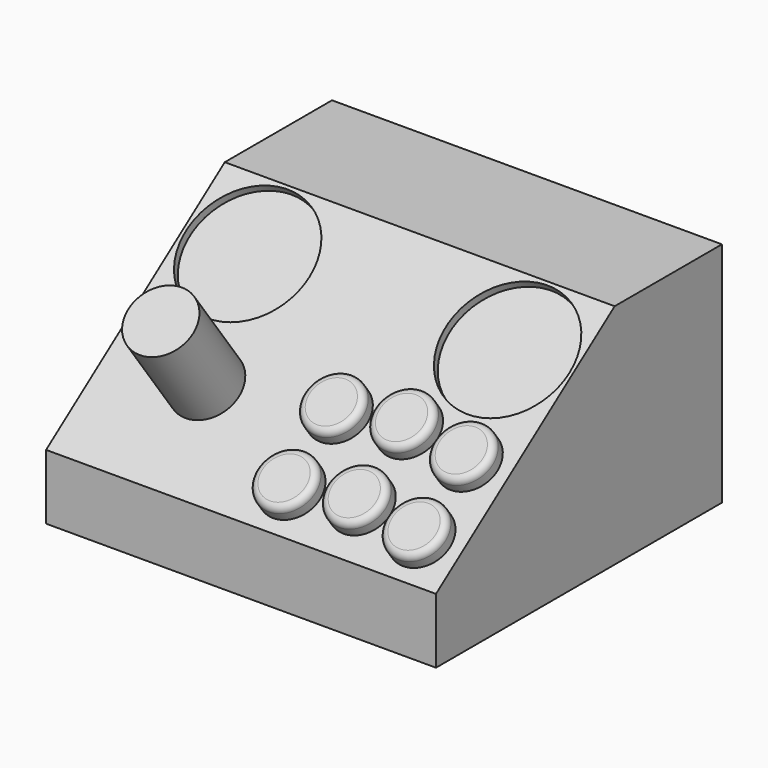
from build123d import *

# Parameters (mm, degrees)
F0_W     = 82.5227291513
F0_H     = 100
F1_DEPTH = 120
F2_R     = 38.1
F3_DEPTH = 5
F4_DEPTH = 5
F2_R_2   = 17.5
F5_DEPTH = 10
F6_DEPTH = 10
F2_R_3   = 20
F7_DEPTH = 60
F8_R     = 4
F9_R     = 4


# Not quite as in the source:
# - the program builds the solid bodies; features that only make, move or delete a surface that nothing else refers to are left out


with BuildPart() as f1:
    # F0 (on Right) → F1 (new body, symmetric)
    with BuildSketch(Plane.YZ):
        Polygon((27.4772708487, -50), (27.4772708487, 50), (-110, -50), align=None)
        with Locations((68.7386354243, 0)):
            Rectangle(F0_W, F0_H)
        Polygon((27.4772708487, -50), (-110, -50), (-110, -90), (110, -90), (110, -50), align=None)
    extrude(amount=F1_DEPTH, both=True)

    # F2 (on face) → F3 (cut)
    with BuildSketch(Plane(origin=(0, -14.2772887805, 19.6280269666), x_dir=(1, 0, 0), z_dir=(0, -0.5882352941, 0.8086898285))):
        with Locations((-80, 11.6323541567)):
            Circle(F2_R)
    extrude(amount=-F3_DEPTH, mode=Mode.SUBTRACT)

    # F2 (on face) → F4 (cut)
    with BuildSketch(Plane(origin=(0, -14.2772887805, 19.6280269666), x_dir=(1, 0, 0), z_dir=(0, -0.5882352941, 0.8086898285))):
        with Locations((80, 11.6323541567)):
            Circle(F2_R)
    extrude(amount=-F4_DEPTH, mode=Mode.SUBTRACT)

    # F2 (on face) → F5 (join)
    with BuildSketch(Plane(origin=(0, -14.2772887805, 19.6280269666), x_dir=(1, 0, 0), z_dir=(0, -0.5882352941, 0.8086898285))):
        with Locations((15, -48.3676458433)):
            Circle(F2_R_2)
    extrude(amount=F5_DEPTH)

    # F2 (on face) → F6 (join)
    with BuildSketch(Plane(origin=(0, -14.2772887805, 19.6280269666), x_dir=(1, 0, 0), z_dir=(0, -0.5882352941, 0.8086898285))):
        with Locations((15, -93.3676458433)):
            Circle(F2_R_2)
        with Locations((55, -43.3676458433)):
            Circle(F2_R_2)
        with Locations((55, -88.3676458433)):
            Circle(F2_R_2)
        with Locations((95, -48.3676458433)):
            Circle(F2_R_2)
        with Locations((95, -93.3676458433)):
            Circle(F2_R_2)
    extrude(amount=F6_DEPTH)

    # F2 (on face) → F7 (join)
    with BuildSketch(Plane(origin=(0, -14.2772887805, 19.6280269666), x_dir=(1, 0, 0), z_dir=(0, -0.5882352941, 0.8086898285))):
        with Locations((-60, -58.3676458433)):
            Circle(F2_R_3)
    extrude(amount=F7_DEPTH)

    # F8
    f8_edges = [f1.edges().sort_by_distance(p)[0] for p in [
        (-2.5, -59.274065, -0.736631),
    ]]
    fillet(f8_edges, radius=F8_R)

    # F9
    f9_edges = [f1.edges().sort_by_distance(p)[0] for p in [
        (37.5, -55.230616, 2.204545),
        (77.5, -59.274065, -0.736631),
        (77.5, -95.665107, -27.207219),
        (37.5, -91.621658, -24.266043),
        (-2.5, -95.665107, -27.207219),
    ]]
    fillet(f9_edges, radius=F9_R)


solid = f1.part
